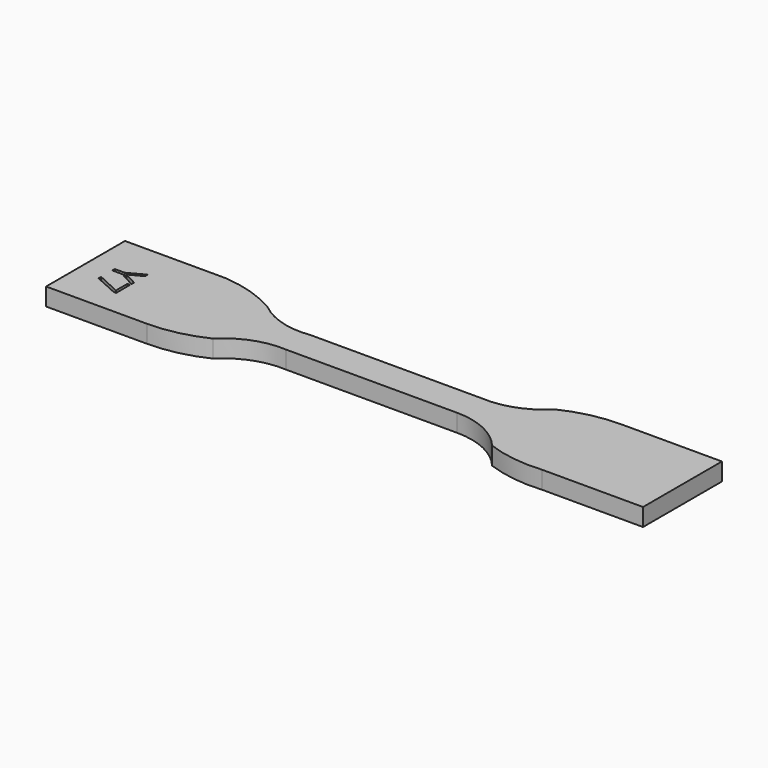
from build123d import *

# Parameters (mm, degrees)
F1_DEPTH     = 3.4
F2_TEXT_SIZE = 7.0564552314
F3_DEPTH     = 1


# Not quite as in the source:
# - Text() gives the source's letters only with a copy of the font that has no kerning and outlines rounded to 1/6400 em; it was checked with that copy


with BuildPart() as f1:
    # F0 (on Top) → F1 (new body)
    with BuildSketch(Plane.XY):
        with BuildLine():
            Line((-14.4320548165, 19.7811394548), (-33.8720548165, 19.7811394548))
            Line((-33.8720548165, 19.7811394548), (-33.8720548165, 0.7811394548))
            Line((-33.8720548165, 0.7811394548), (-14.4320548165, 0.7811394548))
            ThreePointArc((-14.4320548165, 0.7811394548), (-8.9053122052, 1.3996892086), (-3.6520548165, 3.2247301661))
            ThreePointArc((-3.6520548165, 3.2247301661), (1.3014698263, 6.4128780055), (7.1279451835, 7.2811394548))
            Line((7.1279451835, 7.2811394548), (40.1279451835, 7.2811394548))
            ThreePointArc((40.1279451835, 7.2811394548), (46.0837574042, 5.9511158081), (50.9079451835, 2.2137538538))
            ThreePointArc((50.9079451835, 2.2137538538), (56.2191047011, 0.9041953221), (61.6879451835, 0.7811394548))
            Line((61.6879451835, 0.7811394548), (81.1279451835, 0.7811394548))
            Line((81.1279451835, 0.7811394548), (81.1279451835, 19.7811394548))
            Line((81.1279451835, 19.7811394548), (61.6879451835, 19.7811394548))
            ThreePointArc((61.6879451835, 19.7811394548), (56.1612025723, 19.162589701), (50.9079451835, 17.3375487435))
            ThreePointArc((50.9079451835, 17.3375487435), (45.9544205407, 14.1494009041), (40.1279451835, 13.2811394548))
            Line((40.1279451835, 13.2811394548), (7.1279451835, 13.2811394548))
            ThreePointArc((7.1279451835, 13.2811394548), (1.4167452884, 13.6925537245), (-3.6520548165, 16.3560723447))
            ThreePointArc((-3.6520548165, 16.3560723447), (-8.8458057958, 18.686276846), (-14.4320548165, 19.7811394548))
        make_face()
    extrude(amount=F1_DEPTH)

    # F2 (on face) → F3 (cut)
    with BuildSketch(Plane.XY.offset(3.4)):
        with Locations(Location((-29.3720550835, 13.353464842), (0, 0, -90))):
            Text('Y7', F2_TEXT_SIZE, font='Open Sans', text_align=(TextAlign.LEFT, TextAlign.BOTTOM))
    extrude(amount=-F3_DEPTH, mode=Mode.SUBTRACT)


solid = f1.part
